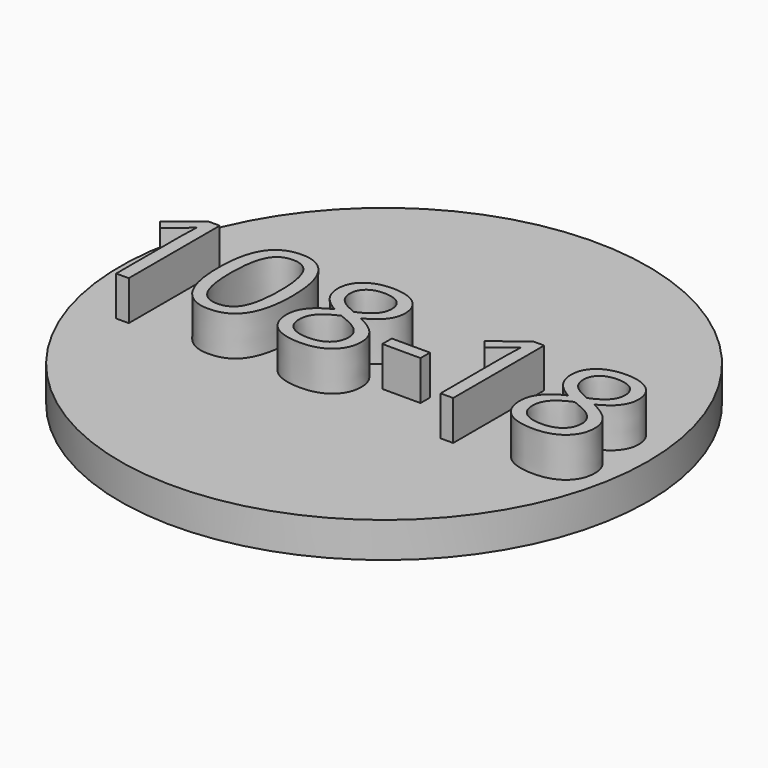
from build123d import *

# Parameters (mm, degrees)
F0_R         = 77.8466159258
F1_DEPTH     = 10.414
F2_TEXT_SIZE = 46.9708031936
F3_DEPTH     = 11.684


# Not quite as in the source:
# - Text() gives the source's letters only with a copy of the font that has no kerning and outlines rounded to 1/6400 em; it was checked with that copy


with BuildPart() as f1:
    # F0 (on Top) → F1 (new body)
    with BuildSketch(Plane.XY):
        with Locations((0, 0.5042813718)):
            Circle(F0_R)
    extrude(amount=F1_DEPTH)

    # F2 (on face) → F3 (join)
    with BuildSketch(Plane.XY.offset(10.414)):
        with Locations((-74.9991621618, -20.3576764973)):
            Text('108-18', F2_TEXT_SIZE, font='Open Sans', text_align=(TextAlign.LEFT, TextAlign.BOTTOM))
    extrude(amount=F3_DEPTH)


solid = f1.part
